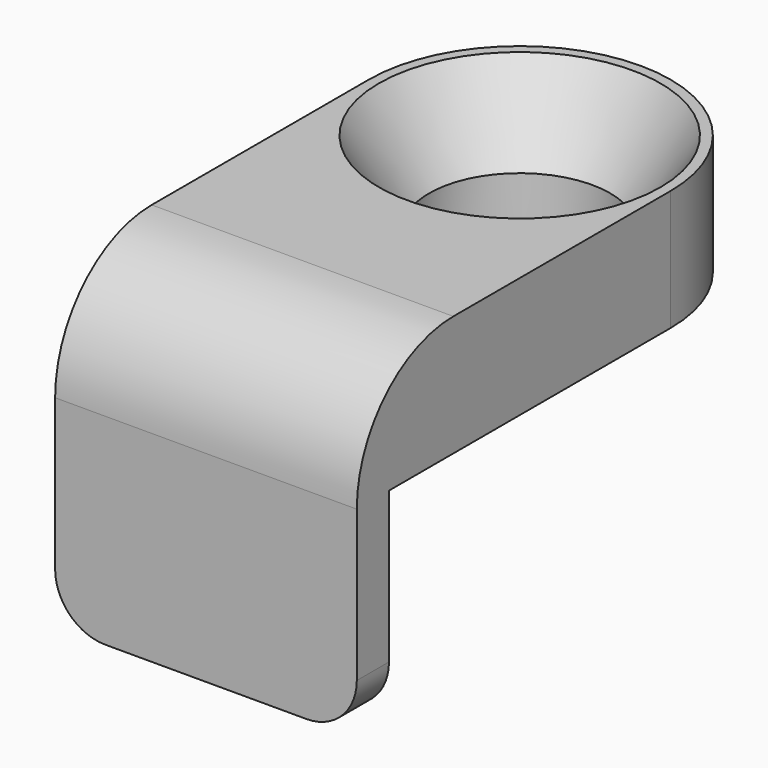
from build123d import *

# Parameters (mm, degrees)
F0_R     = 12
F0_W     = 30
F0_H     = 4
F0_R_2   = 9
F1_DEPTH = 3
F2_DEPTH = 20
F3_DEPTH = 6
F4_SIZE  = 2.99999
F6_DEPTH = 12
F7_SIZE2 = 5
F7_SIZE  = 8
F8_DEPTH = 4
F9_R     = 12
F10_R    = 5


# Not quite as in the source:
# - a fillet or chamfer is up to 0.001 mm smaller than in the source, because OpenCascade refuses the exact size


with BuildPart() as f1:
    # F0 (on Top) → F1 (new body)
    with BuildSketch(Plane.XY):
        with BuildLine():
            Line((15, -35), (15, 0))
            ThreePointArc((15, 0), (0, 15), (-15, 0))
            Line((-15, 0), (-15, -35))
            Line((-15, -35), (15, -35))
        make_face()
        Circle(F0_R, mode=Mode.SUBTRACT)
        with Locations((0, -37)):
            Rectangle(F0_W, F0_H)
        Circle(F0_R)
        Circle(F0_R_2, mode=Mode.SUBTRACT)
    extrude(amount=F1_DEPTH)

    # F0 (on Top) → F2 (join)
    with BuildSketch(Plane.XY):
        with Locations((0, -37)):
            Rectangle(F0_W, F0_H)
    extrude(amount=-F2_DEPTH)

    # F0 (on Top) → F3 (join)
    with BuildSketch(Plane.XY):
        Circle(F0_R)
        Circle(F0_R_2, mode=Mode.SUBTRACT)
    extrude(amount=F3_DEPTH)

    # F4 (size 3 in the source; OpenCascade refuses exactly that, so slightly less here)
    f4_edges = [f1.edges().sort_by_distance(p)[0] for p in [
        (-12, 0, 3),
    ]]
    chamfer(f4_edges, length=F4_SIZE)

    # F0 (on Top) → F6 (join)
    with BuildSketch(Plane.XY):
        with BuildLine():
            Line((15, -35), (15, 0))
            ThreePointArc((15, 0), (0, 15), (-15, 0))
            Line((-15, 0), (-15, -35))
            Line((-15, -35), (15, -35))
        make_face()
        Circle(F0_R, mode=Mode.SUBTRACT)
        Circle(F0_R)
        Circle(F0_R_2, mode=Mode.SUBTRACT)
    extrude(amount=F6_DEPTH)

    # F7
    f7_edges = [f1.edges().sort_by_distance(p)[0] for p in [
        (-9, 0, 12),
    ]]
    f7_side = f1.faces().sort_by_distance((-9, 0, 6))[0]
    chamfer(f7_edges, length=F7_SIZE, length2=F7_SIZE2, reference=f7_side)

    # F8 (add, through all): a face of the model
    f8_faces = [f1.faces().sort_by_distance(p)[0] for p in [
        (0, -35, 7.5),
    ]]
    extrude(f8_faces, amount=F8_DEPTH)

    # F9
    f9_edges = [f1.edges().sort_by_distance(p)[0] for p in [
        (0, -39, 12),
    ]]
    fillet(f9_edges, radius=F9_R)

    # F10
    f10_edges = [f1.edges().sort_by_distance(p)[0] for p in [
        (-15, -37, -20),
        (15, -37, -20),
    ]]
    fillet(f10_edges, radius=F10_R)


solid = f1.part
